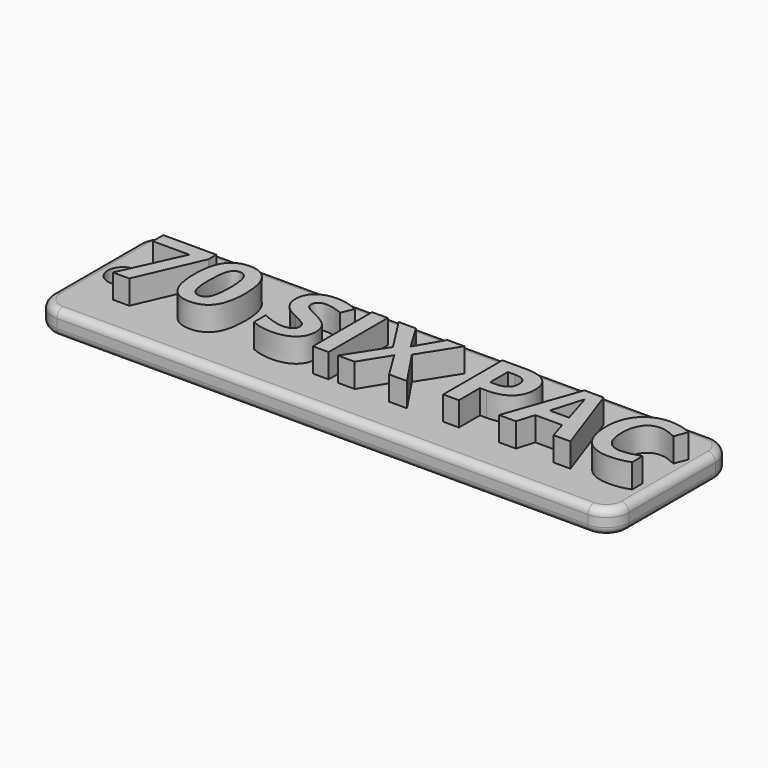
from build123d import *

# Parameters (mm, degrees)
F0_R         = 2
F2_DEPTH     = 3.175
F1_TEXT_SIZE = 13.6900866218
F3_DEPTH     = 6.35
F4_R         = 1
F5_R         = 1


# Not quite as in the source:
# - Text() gives the source's letters only with a copy of the font that has no kerning and outlines rounded to 1/6400 em; it was checked with that copy


with BuildPart() as f2:
    # F0 (on Top) → F2 (new body)
    with BuildSketch(Plane.XY):
        with BuildLine():
            ThreePointArc((38.1, 7.16), (37.2213203436, 9.2813203436), (35.1, 10.16))
            Line((35.1, 10.16), (-35.1, 10.16))
            ThreePointArc((-35.1, 10.16), (-37.2213203436, 9.2813203436), (-38.1, 7.16))
            Line((-38.1, 7.16), (-38.1, -7.16))
            ThreePointArc((-38.1, -7.16), (-37.2213203436, -9.2813203436), (-35.1, -10.16))
            Line((-35.1, -10.16), (35.1, -10.16))
            ThreePointArc((35.1, -10.16), (37.2213203436, -9.2813203436), (38.1, -7.16))
            Line((38.1, -7.16), (38.1, 7.16))
        make_face()
        with Locations((-34.5066972077, 0)):
            Circle(F0_R, mode=Mode.SUBTRACT)
    extrude(amount=F2_DEPTH)

    # F1 (on Top) → F3 (join)
    with BuildSketch(Plane.XY):
        with Locations((-33.528, -4.7768623677)):
            Text('70 SIX PAC', F1_TEXT_SIZE, font='Open Sans', font_style=FontStyle.BOLD, text_align=(TextAlign.LEFT, TextAlign.BOTTOM))
    extrude(amount=F3_DEPTH)

    # F4
    f4_edges = [f2.edges().sort_by_distance(p)[0] for p in [
        (0, 10.16, 3.175),
    ]]
    fillet(f4_edges, radius=F4_R)

    # F5
    f5_edges = [f2.edges().sort_by_distance(p)[0] for p in [
        (0, 10.16, 0),
    ]]
    fillet(f5_edges, radius=F5_R)


solid = f2.part
